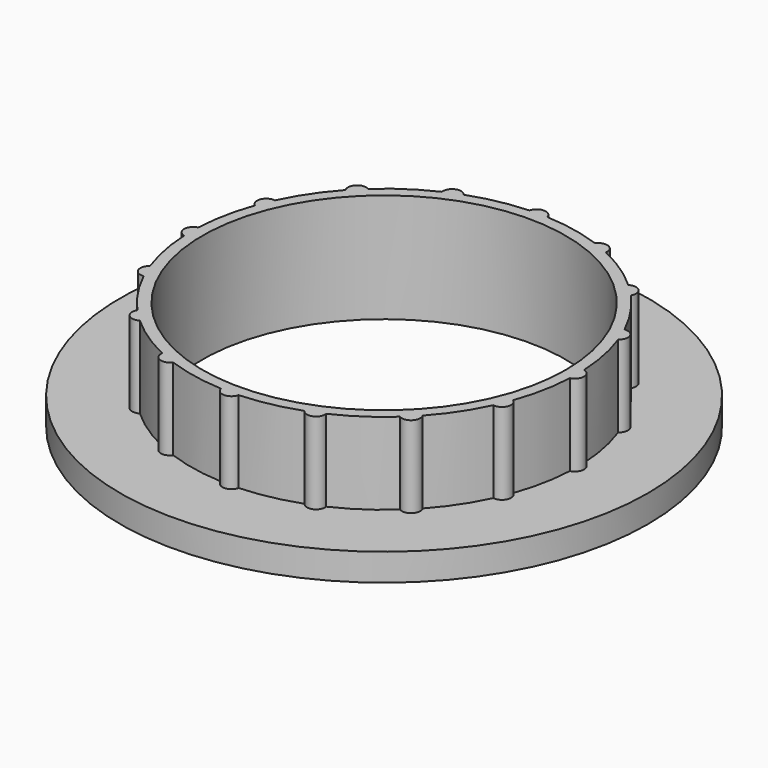
from build123d import *

# Parameters (mm, degrees)
F3_DEPTH        = 9
F3_COPIES_COUNT = 16


# Not quite as in the source:
# - a pattern or mirror of a feature is missing from the dataset's text; its kind, count and spacing are read off the source's solid


with BuildPart() as f1:
    # F0 (on Front) → F1 (revolve)
    with BuildSketch(Plane.XZ):
        Polygon((20, 12), (20, 0), (29.0510931471, 0), (29.0510931471, 3), (21.25, 3), (21.25, 12), align=None)
    revolve(axis=Axis((0, 0, 7.2627740937), (0, 0, 1)))

    # F2 (on face) → F3 (join, through all)
    with BuildSketch(Plane.XY.offset(3)):
        with BuildLine():
            ThreePointArc((-0.9737363442, 21.2276785714), (0, 21.25), (0.9737363442, 21.2276785714))
            ThreePointArc((0.9737363442, 21.2276785714), (0, 22), (-0.9737363442, 21.2276785714))
        make_face()
    f3 = extrude(amount=F3_DEPTH)

    # F3_copies: F3 ×16 about axis
    f3_copies_axis = Axis((0, 0, 0), (0, 0, 1))
    for i in range(1, F3_COPIES_COUNT):
        add(f3.rotate(f3_copies_axis, i * 360 / F3_COPIES_COUNT))


solid = f1.part
